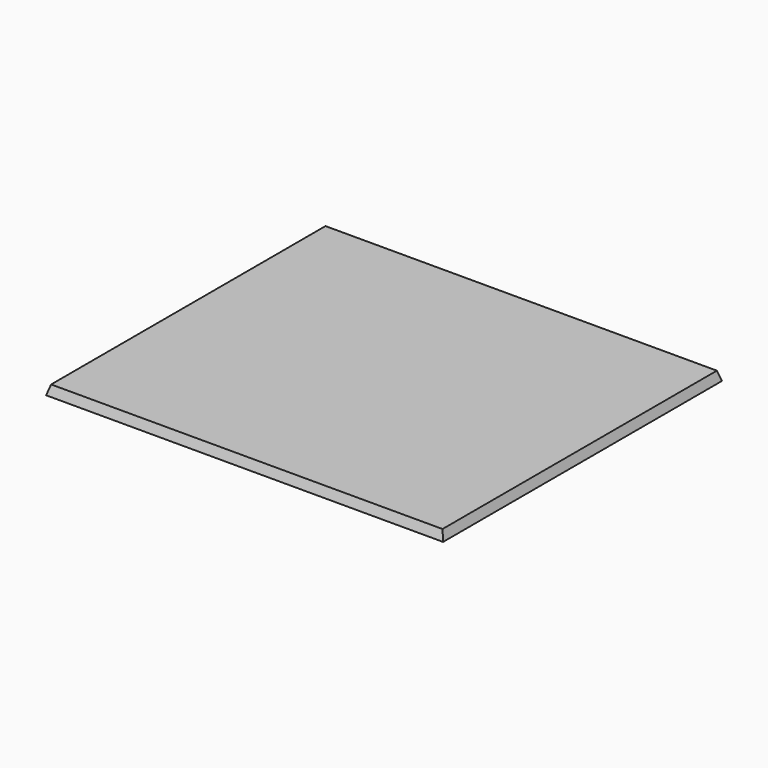
from build123d import *

# Parameters (mm, degrees)
F0_W        = 108
F0_H        = 95
F1_DEPTH    = 2.5
F2_T1_DEPTH = 133.959416678
F2_T3_DEPTH = 120.959416678


# Not quite as in the source:
# - a fillet or chamfer that OpenCascade refuses, or shapes differently, is made with other operations: its cross-section is extruded or revolved along the edge and cut away or added


with BuildPart() as f1:
    # F0 (on Top) → F1 (new body)
    with BuildSketch(Plane.XY):
        Rectangle(F0_W, F0_H)
    extrude(amount=F1_DEPTH)

    # F2: chamfer of 5 x 1.5 on 4 edges, made by hand

    # F2_s2 → F2_t1 (cut)
    with BuildSketch(Plane.YZ.offset(-66.979708339)):
        Polygon((-47.5, -2.5), (-46, 2.5), (-47.5, 2.5), align=None)
        Polygon((47.5, -2.5), (46, 2.5), (47.5, 2.5), align=None)
    extrude(amount=F2_T1_DEPTH, mode=Mode.SUBTRACT)

    # F2_s4 → F2_t3 (cut)
    with BuildSketch(Plane.XZ.offset(-60.479708339)):
        Polygon((-54, -2.5), (-52.5, 2.5), (-54, 2.5), align=None)
        Polygon((54, -2.5), (52.5, 2.5), (54, 2.5), align=None)
    extrude(amount=F2_T3_DEPTH, mode=Mode.SUBTRACT)


solid = f1.part
